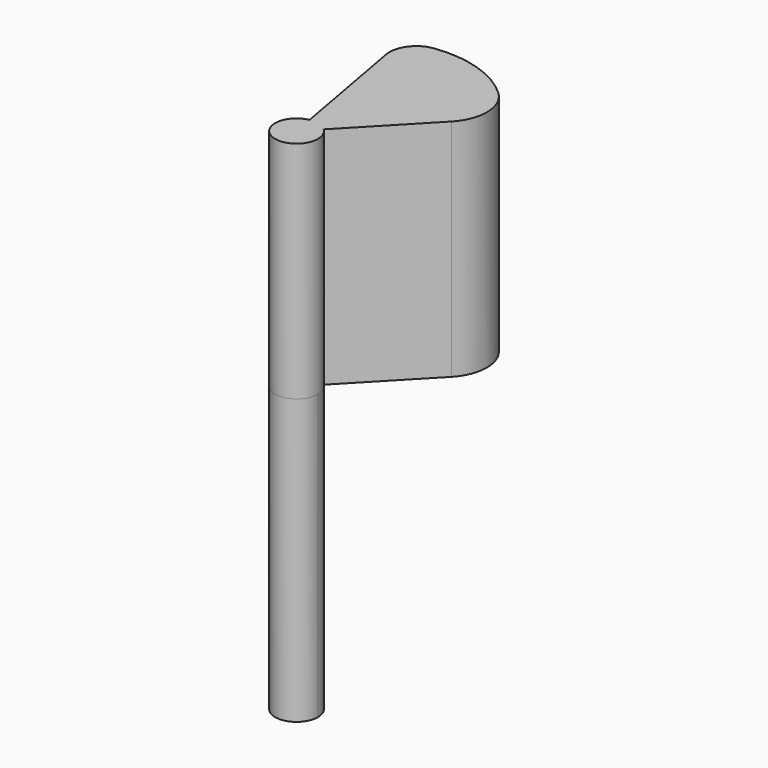
from build123d import *
from build123d import SkipClean  # not in build123d's __all__

# Parameters (mm, degrees)
F1_DEPTH = 105.1
F3_DEPTH = 132.9


with BuildPart() as f1:
    # F0 (on Top) → F1 (new body)
    with BuildSketch(Plane.XY):
        with BuildLine():
            Line((-12.2990868875, 67.7678571429), (-1.7857142857, 9.83926951))
            ThreePointArc((-1.7857142857, 9.83926951), (-2.8810809532, -9.5759789338), (6.9184089901, 7.2204997781))
            Line((6.9184089901, 7.2204997781), (39.4409995563, 41.1631820199))
            ThreePointArc((39.4409995563, 41.1631820199), (44.9882549975, 55.6853190171), (38.4593810195, 69.7934128102))
            ThreePointArc((38.4593810195, 69.7934128102), (19.8153219741, 80.5054589403), (-1.6036428236, 82.3967064051))
            ThreePointArc((-1.6036428236, 82.3967064051), (-10.0907027029, 77.3775144162), (-12.2990868875, 67.7678571429))
        make_face()
    extrude(amount=F1_DEPTH)

    # F2 (on face) → F3 (join)
    with BuildSketch(Plane.XY):
        with BuildLine():
            ThreePointArc((-1.7857142857, 9.83926951), (-6.4086994446, -7.6764947358), (10, 0))
            ThreePointArc((10, 0), (9.197393378, 3.9252968104), (6.9184089901, 7.2204997781))
            ThreePointArc((6.9184089901, 7.2204997781), (2.8810809532, 9.5759789338), (-1.7857142857, 9.83926951))
        make_face()
    with SkipClean():  # cleaning this boolean's faces spoils the solid; the shape is the same uncleaned
        extrude(amount=-F3_DEPTH)


solid = f1.part
